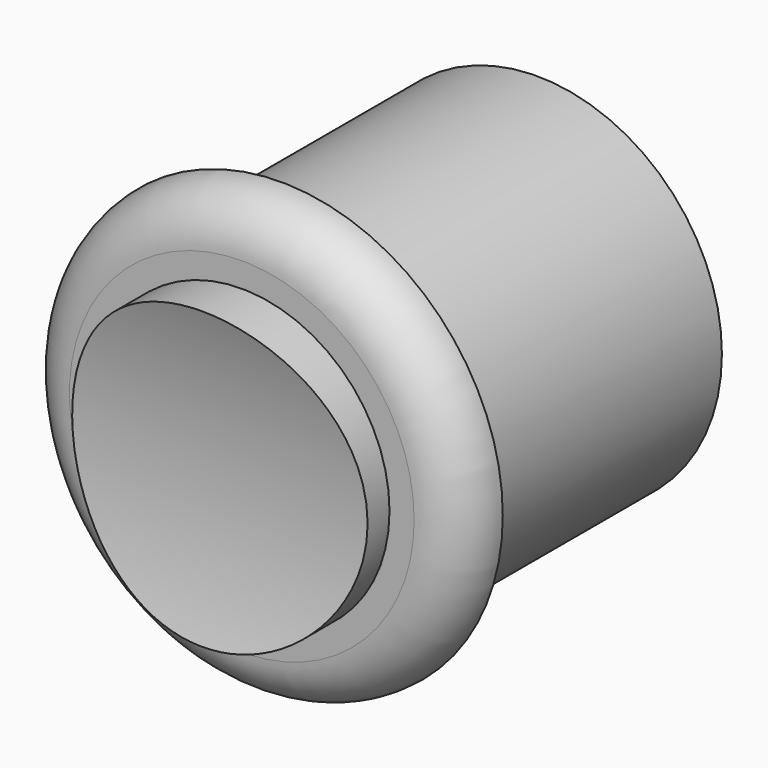
from build123d import *

# Parameters (mm, degrees)
F0_R     = 7.5
F1_DEPTH = 15
F2_R     = 9
F3_DEPTH = 2
F4_R     = 6
F5_DEPTH = 2
F7_DEPTH = 12.5
F8_R     = 1.99999


# Not quite as in the source:
# - a fillet or chamfer is up to 0.001 mm smaller than in the source, because OpenCascade refuses the exact size


with BuildPart() as f1:
    # F0 (on Front) → F1 (new body)
    with BuildSketch(Plane.XZ):
        Circle(F0_R)
    extrude(amount=-F1_DEPTH)

    # F2 (on Front) → F3 (join)
    with BuildSketch(Plane.XZ):
        Circle(F2_R)
    extrude(amount=-F3_DEPTH)

    # F4 (on Front) → F5 (join)
    with BuildSketch(Plane.XZ):
        Circle(F4_R)
    extrude(amount=F5_DEPTH)

    # F6 (on Right) → F7 (cut, symmetric)
    with BuildSketch(Plane.YZ):
        with BuildLine():
            ThreePointArc((-2, -6), (-1.1103724444, 0), (-2, 6))
            Line((-2, 6), (-2, -6))
        make_face()
    extrude(amount=F7_DEPTH, both=True, mode=Mode.SUBTRACT)

    # F8 (radius 2 in the source; OpenCascade refuses exactly that, so slightly less here)
    f8_edges = [f1.edges().sort_by_distance(p)[0] for p in [
        (-9, 0, 0),
    ]]
    fillet(f8_edges, radius=F8_R)


solid = f1.part
